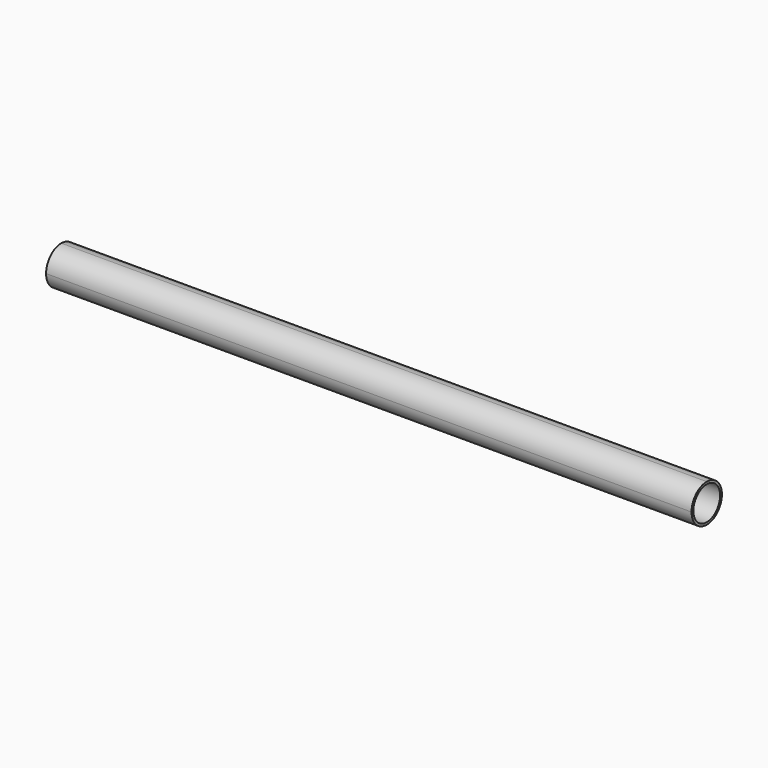
from build123d import *

# Parameters (mm, degrees)
F1_DEPTH = 25
F2_R     = 24.99999
F4_D     = 44
F4_DEPTH = 403.0937720853
F6_D     = 44


# Not quite as in the source:
# - a fillet or chamfer is up to 0.001 mm smaller than in the source, because OpenCascade refuses the exact size


with BuildPart() as f1:
    # F0 (on Top) → F1 (new body, symmetric)
    with BuildSketch(Plane.XY):
        Polygon((446.9072279147, 0), (0, 0), (-403.0927720853, 0), (-403.0927720853, -25), (446.9072279147, -25), align=None)
        Polygon((-403.0927720853, 0), (0, 0), (446.9072279147, 0), (446.9072279147, 25), (-403.0927720853, 25), align=None)
    extrude(amount=F1_DEPTH, both=True)

    # F2 (radius 25 in the source; OpenCascade refuses exactly that, so slightly less here)
    f2_edges = [f1.edges().sort_by_distance(p)[0] for p in [
        (21.907228, -25, -25),
        (21.907228, 25, -25),
        (21.907228, 25, 25),
        (21.907228, -25, 25),
    ]]
    fillet(f2_edges, radius=F2_R)

    # F4 (through all, one way)
    with BuildSketch(Plane.YZ):
        with Locations((0, 0)):
            Circle(F4_D / 2)
    extrude(amount=-F4_DEPTH, mode=Mode.SUBTRACT)

    # F6 (through all)
    with Locations(Plane.YZ.offset(446.9072279147)):
        with Locations((0, 0)):
            Hole(F6_D / 2)


solid = f1.part
